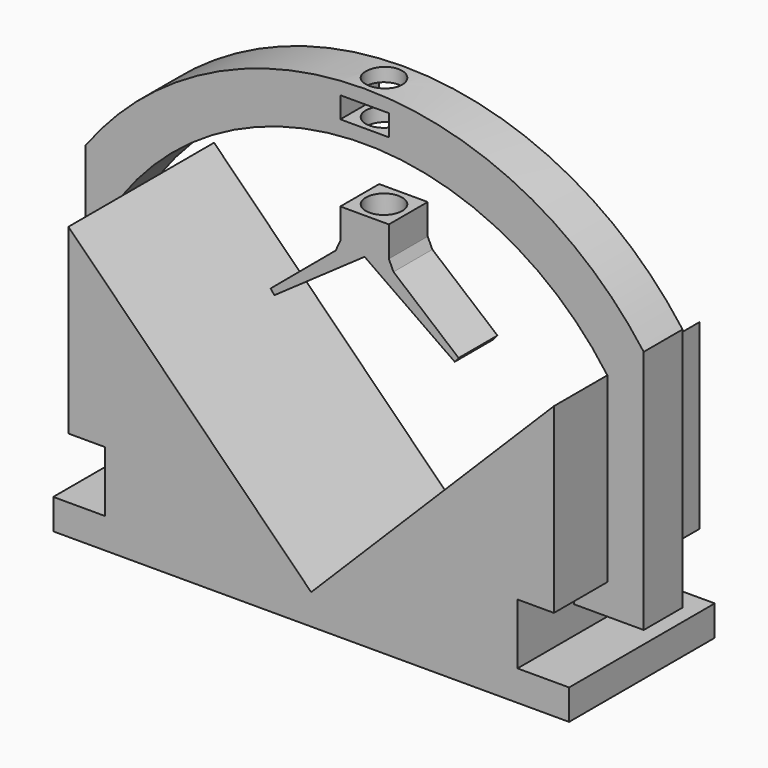
from build123d import *

# Parameters (mm, degrees)
F0_W      = 85
F0_H      = 30
F1_DEPTH  = 5
F3_DEPTH  = 15
F5_DEPTH  = 4
F6_R      = 3
F7_DEPTH  = 80
F9_DEPTH  = 4
F10_R     = 3
F11_DEPTH = 5
F12_SIZE  = 1


with BuildPart() as f1:
    # F0 (on Top) → F1 (new body)
    with BuildSketch(Plane.XY):
        Rectangle(F0_W, F0_H)
    extrude(amount=-F1_DEPTH)

    # F2 (on Front) → F3 (join, symmetric)
    with BuildSketch(Plane.XZ):
        Polygon((-34, 0), (0, 0), (-40, 40), (-40, 10), (-34, 10), align=None)
        Polygon((40, 40), (0, 0), (34, 0), (34, 10), (40, 10), align=None)
    extrude(amount=F3_DEPTH, both=True)


with BuildPart() as f5:
    # F4 (on Front) → F5 (new body, symmetric)
    with BuildSketch(Plane.XZ):
        with BuildLine():
            Line((-40, 10), (-40, 40))
            ThreePointArc((-40, 40), (-22.4891657332, 55.1249006818), (0, 60.5681866361))
            ThreePointArc((0, 60.5681866361), (22.4891657332, 55.1249006818), (40, 40))
            Line((40, 40), (40, 10))
            Line((40, 10), (34.5, 10))
            Line((34.5, 10), (34.5, 5))
            Line((34.5, 5), (46, 5))
            Line((46, 5), (46, 45.3515663186))
            ThreePointArc((46, 45.3515663186), (25.7634016531, 62.4351125068), (0, 68.5681866361))
            ThreePointArc((0, 68.5681866361), (-25.7634016531, 62.4351125068), (-46, 45.3515663186))
            Line((-46, 45.3515663186), (-46, 5))
            Line((-46, 5), (-34.5, 5))
            Line((-34.5, 5), (-34.5, 10))
            Line((-34.5, 10), (-40, 10))
        make_face()
        Polygon((-4, 66.3181866361), (0, 66.3181866361), (4, 66.3181866361), (4, 62.8181866361), (0, 62.8181866361), (-4, 62.8181866361), align=None, mode=Mode.SUBTRACT)
    extrude(amount=F5_DEPTH, both=True)

    # F6 (on Top) → F7 (cut)
    with BuildSketch(Plane.XY):
        Circle(F6_R)
    extrude(amount=F7_DEPTH, mode=Mode.SUBTRACT)


with BuildPart() as f9:
    # F8 (on Front) → F9 (new body, symmetric)
    with BuildSketch(Plane.XZ):
        Polygon((4, 50.1803820431), (0, 50.1803820431), (-4, 50.1803820431), (-4, 44.1803820431), (-15.4966514918, 34.5457048573), (-14.8543396794, 33.7792614245), (0, 44.1803820431), (14.8543396794, 33.7792614245), (15.4966514918, 34.5457048573), (4, 44.1803820431), align=None)
    extrude(amount=F9_DEPTH, both=True)

    # F10 (on face) → F11 (cut)
    with BuildSketch(Plane.XY.offset(50.1803820431)):
        Circle(F10_R)
    extrude(amount=-F11_DEPTH, mode=Mode.SUBTRACT)

    # F12
    f12_edges = [f9.edges().sort_by_distance(p)[0] for p in [
        (-4, 0, 44.180382),
        (4, 0, 44.180382),
    ]]
    chamfer(f12_edges, length=F12_SIZE)


solid = Compound([f1.part, f5.part, f9.part])
